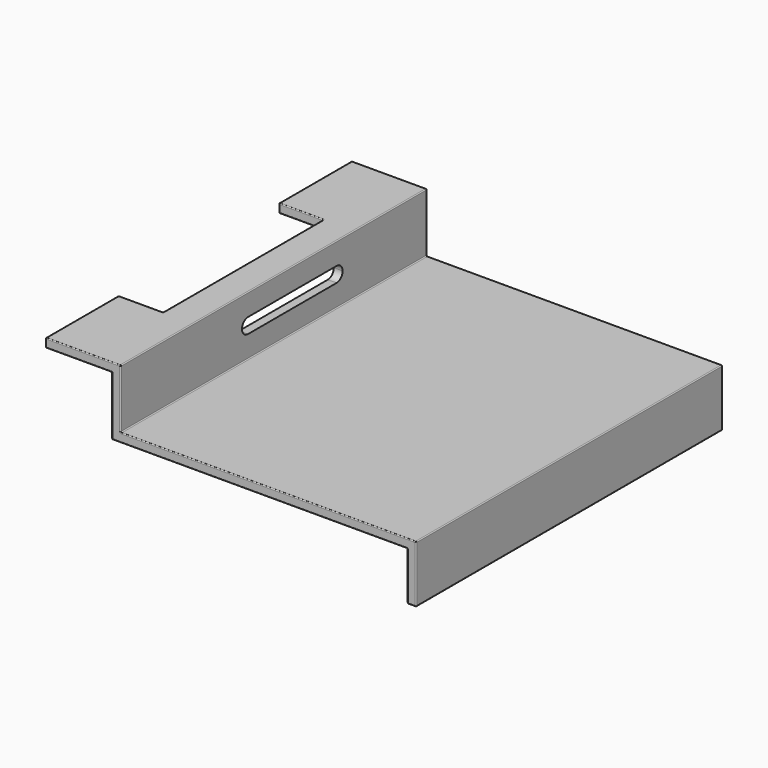
from build123d import *

# Parameters (mm, degrees)
F1_DEPTH = 434
F2_W     = 50.4274696951
F2_H     = 227
F3_DEPTH = 132.001
F5_DEPTH = 25.4
F6_R     = 1


with BuildPart() as f1:
    # F0 (on Front) → F1 (new body)
    with BuildSketch(Plane.XZ):
        Polygon((-133.9674020287, 67), (-218.9674020287, 67), (-218.9674020287, 57), (-143.9674020287, 57), (-143.9674020287, -10), (191.0325979713, -10), (191.0325979713, -65), (201.0325979713, -65), (201.0325979713, 0), (-133.9674020287, 0), align=None)
    extrude(amount=F1_DEPTH)

    # F2 (on face) → F3 (cut, through all)
    with BuildSketch(Plane.XY.offset(67)):
        with Locations((-193.7536671811, -217)):
            Rectangle(F2_W, F2_H)
    extrude(amount=-F3_DEPTH, mode=Mode.SUBTRACT)

    # F4 (on face) → F5 (cut)
    with BuildSketch(Plane.YZ.offset(-133.9674020287)):
        with BuildLine():
            Line((-127.8944141269, 42), (-253.5, 42))
            ThreePointArc((-253.5, 42), (-259.5104076401, 39.5104076401), (-262, 33.5))
            ThreePointArc((-262, 33.5), (-259.5104076401, 27.4895923599), (-253.5, 25))
            Line((-253.5, 25), (-127.8944141269, 25))
            ThreePointArc((-127.8944141269, 25), (-121.8840064868, 27.4895923599), (-119.3944141269, 33.5))
            ThreePointArc((-119.3944141269, 33.5), (-121.8840064868, 39.5104076401), (-127.8944141269, 42))
        make_face()
    extrude(amount=-F5_DEPTH, mode=Mode.SUBTRACT)

    # F6
    f6_edges = [f1.edges().sort_by_distance(p)[0] for p in [
        (-193.753667, -103.5, 67),
        (-168.539932, -103.5, 62),
        (-168.539932, -217, 57),
        (-168.539932, -217, 67),
        (-218.967402, -51.75, 67),
        (-218.967402, -51.75, 57),
        (-218.967402, -103.5, 62),
        (-218.967402, 0, 62),
        (-176.467402, 0, 67),
        (-133.967402, -217, 67),
        (-218.967402, -382.25, 67),
        (-218.967402, -382.25, 57),
        (-218.967402, -330.5, 62),
        (-193.753667, -330.5, 57),
        (-193.753667, -330.5, 67),
        (-168.539932, -330.5, 62),
        (-176.467402, -434, 67),
        (-218.967402, -434, 62),
        (-181.467402, -434, 57),
        (-143.967402, -434, 23.5),
        (-133.967402, -434, 33.5),
        (-143.967402, -217, -10),
        (-143.967402, 0, 23.5),
        (-133.967402, 0, 33.5),
        (33.532598, 0, 0),
        (23.532598, 0, -10),
        (-181.467402, 0, 57),
        (33.532598, -434, 0),
        (23.532598, -434, -10),
        (-133.967402, -217, 0),
        (201.032598, -217, 0),
        (201.032598, -434, -32.5),
        (191.032598, -434, -37.5),
        (196.032598, -434, -65),
        (201.032598, -217, -65),
        (191.032598, -217, -65),
        (201.032598, 0, -32.5),
        (191.032598, 0, -37.5),
        (191.032598, -217, -10),
        (-193.753667, -103.5, 57),
    ]]
    fillet(f6_edges, radius=F6_R)


solid = f1.part
